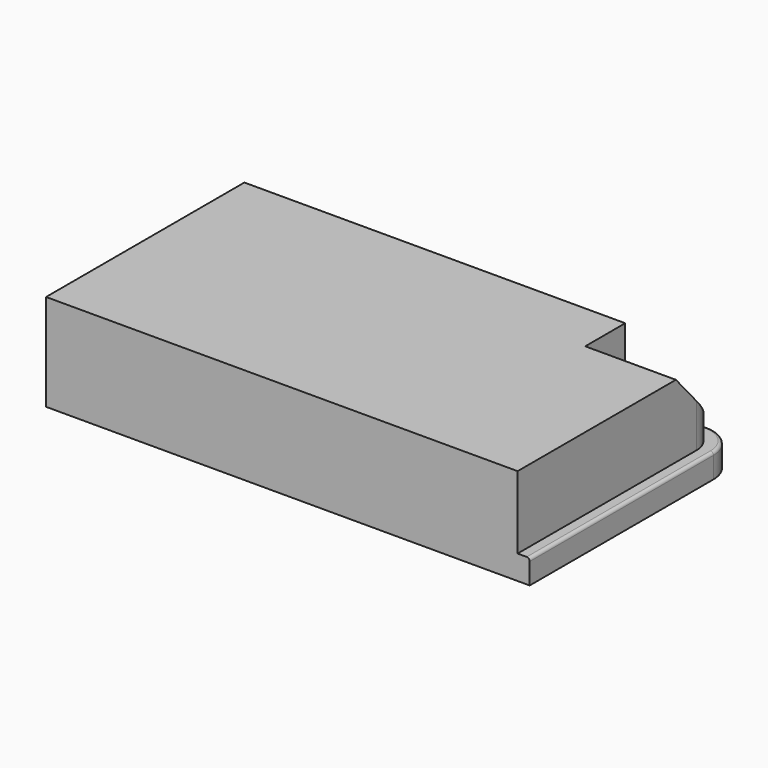
from build123d import *

# Parameters (mm, degrees)
F0_W     = 80
F0_H     = 43
F1_DEPTH = 4
F2_W     = 78
F2_H     = 41
F3_DEPTH = 12
F4_R     = 5
F5_R     = 0.5
F7_DEPTH = 15
F8_R     = 4


# Not quite as in the source:
# - a feature of the source that left no trace in its solid (it failed there, or was rolled back) is left out


with BuildPart() as f1:
    # F0 (on Top) → F1 (new body)
    with BuildSketch(Plane.XY):
        with Locations((40, 21.5)):
            Rectangle(F0_W, F0_H)
    extrude(amount=F1_DEPTH)

    # F2 (on face) → F3 (join)
    with BuildSketch(Plane.XY.offset(4)):
        with Locations((39, 20.5)):
            Rectangle(F2_W, F2_H)
    extrude(amount=F3_DEPTH)

    # F4
    f4_edges = [f1.edges().sort_by_distance(p)[0] for p in [
        (80, 43, 2),
    ]]
    fillet(f4_edges, radius=F4_R)

    # F5
    f5_edges = [f1.edges().sort_by_distance(p)[0] for p in [
        (37.5, 43, 4),
        (78.535534, 41.535534, 4),
        (80, 19, 4),
    ]]
    fillet(f5_edges, radius=F5_R)

    # F6 (on face) → F7 (cut)
    with BuildSketch(Plane.YZ.offset(78)):
        Polygon((41, 16), (32.7275320888, 16), (41, 6.6185845062), align=None)
    extrude(amount=-F7_DEPTH, mode=Mode.SUBTRACT)

    # F8
    f8_edges = [f1.edges().sort_by_distance(p)[0] for p in [
        (78, 41, 5.309292),
    ]]
    fillet(f8_edges, radius=F8_R)


solid = f1.part
